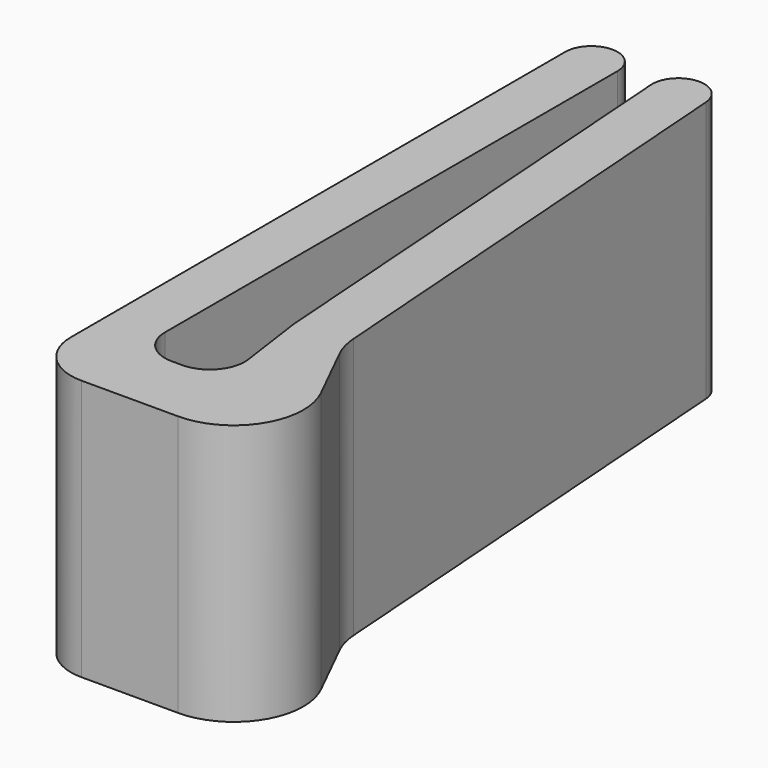
from build123d import *

# Parameters (mm, degrees)
F1_DEPTH = 19.05
F3_DEPTH = 1.27
F3_TAPER = 30


# Not quite as in the source:
# - ends of sketch curves that miss each other by under 0.0002 mm in the source are joined


with BuildPart() as f1:
    # F0 (on Top) → F1 (new body)
    with BuildSketch(Plane.XY):
        with BuildLine():
            Line((0, 48.895), (0, 3.81))
            ThreePointArc((0, 3.81), (1.1159231637, 1.1159231637), (3.81, 0))
            Line((3.81, 0), (10.8694752949, 0))
            ThreePointArc((10.8694752949, 0), (15.1850721495, 2.4000701897), (15.4228204366, 7.3324315794))
            Line((15.4228204366, 7.3324315794), (13.2134093055, 11.7988098401))
            ThreePointArc((13.2134093055, 11.7988098401), (12.8651563088, 12.7167993307), (12.7, 13.684636222))
            Line((12.7, 13.684636222), (10.1424057316, 49.0324769491))
            ThreePointArc((10.1424057316, 49.0324769491), (9.5427497716, 50.2871367633), (8.2501762867, 50.7999840172))
            Line((8.2501762867, 50.7999840172), (8.2423728139, 50.8))
            ThreePointArc((8.2423728139, 50.8), (6.8534050374, 50.1903975816), (6.35, 48.7595199989))
            Line((6.35, 48.7595199989), (8.89, 13.134720074))
            ThreePointArc((8.89, 13.134720074), (8.901535038, 13.0044810095), (8.9175320778, 12.8747144278))
            Line((8.9175320778, 12.8747144278), (9.607234407, 7.973977099))
            ThreePointArc((9.607234407, 7.973977099), (9.009141131, 5.9537920045), (7.092020656, 5.08))
            Line((7.092020656, 5.08), (6.35, 5.08))
            ThreePointArc((6.35, 5.08), (4.5539487758, 5.8239487758), (3.81, 7.62))
            Line((3.81, 7.62), (3.81, 48.895))
            ThreePointArc((3.81, 48.895), (3.2520384182, 50.2420384182), (1.905, 50.8))
            ThreePointArc((1.905, 50.8), (0.5579615818, 50.2420384182), (0, 48.895))
        make_face()
    extrude(amount=F1_DEPTH)


with BuildPart() as f3:
    # F2 (on face) → F3 (new body)
    with BuildSketch(Plane(origin=(0, 0, 0), x_dir=(0, -1, 0), z_dir=(-1, 0, 0))):
        Polygon((-29.6520567884, 11.6832929166), (-23.0529432116, 11.6832929166), (-26.3525, 17.3982929166), align=None)
    extrude(amount=F3_DEPTH, taper=F3_TAPER)


with BuildPart() as f3b:
    # F2 (on face) → F3, piece 2 (new body)
    with BuildSketch(Plane(origin=(0, 0, 0), x_dir=(0, -1, 0), z_dir=(-1, 0, 0))):
        Polygon((-32.9794660211, 5.8412929166), (-26.6065, 5.8412929166), (-29.6799092326, 11.5562929166), align=None)
    extrude(amount=F3_DEPTH, taper=F3_TAPER)


with BuildPart() as f3c:
    # F2 (on face) → F3, piece 3 (new body)
    with BuildSketch(Plane(origin=(0, 0, 0), x_dir=(0, -1, 0), z_dir=(-1, 0, 0))):
        Polygon((-26.3525, 5.8412929166), (-19.7533864232, 5.8412929166), (-23.0529432116, 11.5562929166), align=None)
    extrude(amount=F3_DEPTH, taper=F3_TAPER)


solid = Compound([f1.part, f3.part, f3b.part, f3c.part])
